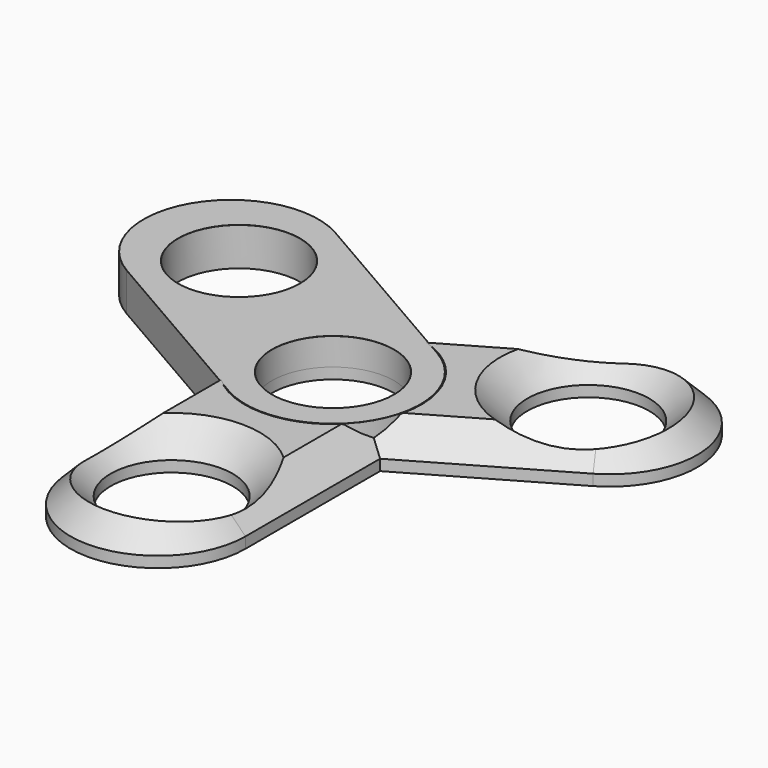
from build123d import *

# Parameters (mm, degrees)
F1_DEPTH    = 7
F2_R        = 11.15
F3_DEPTH    = 7.001
F5_COUNT    = 3
F6_R        = 0.0241421356
F7_T1_DEPTH = 40
F7_T3_DEPTH = 40
F7_T6_ANGLE = 180
F7_T8_ANGLE = 180
F8_T1_DEPTH = 40
F8_T4_ANGLE = 180
F8_T6_ANGLE = 180


# Not quite as in the source:
# - a fillet or chamfer that OpenCascade refuses, or shapes differently, is made with other operations: its cross-section is extruded or revolved along the edge and cut away or added


with BuildPart() as f1:
    # F0 (on Top) → F1 (new body)
    with BuildSketch(Plane.XY):
        with BuildLine():
            ThreePointArc((-16, 0), (0, -16), (16, 0))
            ThreePointArc((16, 0), (0, 16), (-16, 0))
        make_face()
        with BuildLine():
            Line((16, -40), (16, 0))
            ThreePointArc((16, 0), (0, -16), (-16, 0))
            Line((-16, 0), (-16, -40))
            ThreePointArc((-16, -40), (0, -24), (16, -40))
        make_face()
        with BuildLine():
            ThreePointArc((-16, -40), (0, -56), (16, -40))
            ThreePointArc((16, -40), (0, -24), (-16, -40))
        make_face()
    extrude(amount=F1_DEPTH)

    # F2 (on face) → F3 (cut, through all)
    with BuildSketch(Plane.XY.offset(7)):
        Circle(F2_R)
        with Locations((0, -36.8724052611)):
            Circle(F2_R)
    extrude(amount=-F3_DEPTH, mode=Mode.SUBTRACT)


with BuildPart() as f5_1:
    # F5: instance of F1
    add(f1.part.rotate(Axis((0, 0, -10.0436238572), (0, 0, -1)), 1 * 360 / F5_COUNT))

    # F6
    f6_edges = [f5_1.edges().sort_by_distance(p)[0] for p in [
        (-26.641016, 33.856406, 3.5),
        (13.856406, -8, 7),
        (-25.320508, -3.856406, 7),
        (-9.320508, 23.856406, 7),
        (-48.497423, 28, 7),
        (-26.35744, 28.092386, 7),
        (5.575, 9.656183, 7),
        (-42.641016, 6.143594, 3.5),
        (-8, -13.856406, 3.5),
        (-25.320508, -3.856406, 0),
        (-9.320508, 23.856406, 0),
    ]]
    fillet(f6_edges, radius=F6_R)


with BuildPart() as f5_2:
    # F5: instance of F1
    add(f1.part.rotate(Axis((0, 0, -10.0436238572), (0, 0, -1)), 2 * 360 / F5_COUNT))

    # F7: chamfer of 5 on 6 edges, made by hand

    # F7_s2 → F7_t1 (cut)
    with BuildSketch(Plane(origin=(34.6410161514, 20, 0), x_dir=(0, 0, 1), z_dir=(-0.8660254038, -0.5, 0))):
        Polygon((2, 16), (7, 11), (7, 16), align=None)
    extrude(amount=F7_T1_DEPTH, mode=Mode.SUBTRACT)

    # F7_s4 → F7_t3 (cut)
    with BuildSketch(Plane(origin=(0, 0, 0), x_dir=(0, 0, 1), z_dir=(0.8660254038, 0.5, 0))):
        Polygon((2, 16), (7, 11), (7, 16), align=None)
    extrude(amount=F7_T3_DEPTH, mode=Mode.SUBTRACT)

    # F7_s5 → F7_t6 (revolve, cut)
    with BuildSketch(Plane(origin=(0, 0, 0), x_dir=(0, 0, 1), z_dir=(0.8660254038, 0.5, 0))):
        Polygon((2, -16), (7, -11), (7, -16), align=None)
    revolve(axis=Axis((0, 0, 7), (0, 0, 1)), revolution_arc=F7_T6_ANGLE, mode=Mode.SUBTRACT)

    # F7_s7 → F7_t8 (revolve, cut)
    with BuildSketch(Plane(origin=(34.6410161514, 20, 0), x_dir=(0, 0, 1), z_dir=(-0.8660254038, -0.5, 0))):
        Polygon((7, -11), (2, -16), (7, -16), align=None)
    revolve(axis=Axis((34.6410161514, 20, 7), (0, 0, 1)), revolution_arc=F7_T8_ANGLE, mode=Mode.SUBTRACT)

    # F7_s9 → F7_t10 (revolve, cut)
    with BuildSketch(Plane(origin=(31.9324396547, 18.4362026305, 0), x_dir=(0, 0, 1), z_dir=(0.8660254038, 0.5, 0))):
        Polygon((7, -16.15), (2, -11.15), (7, -11.15), align=None)
    revolve(axis=Axis((31.9324396547, 18.4362026305, 7), (0, 0, 1)), mode=Mode.SUBTRACT)

    # F7_s11 → F7_t12 (revolve, cut)
    with BuildSketch(Plane(origin=(0, 0, 0), x_dir=(0, 0, 1), z_dir=(0.8660254038, 0.5, 0))):
        Polygon((7, -16.15), (2, -11.15), (7, -11.15), align=None)
    revolve(axis=Axis((0, 0, 7), (0, 0, 1)), mode=Mode.SUBTRACT)


with BuildPart() as f1_1:
    add(f1.part)

    # F8: chamfer of 5 on 6 edges, made by hand

    # F8_s2 → F8_t1 (cut)
    with BuildSketch(Plane.XZ):
        Polygon((16, 2), (11, 7), (16, 7), align=None)
        Polygon((-16, 2), (-11, 7), (-16, 7), align=None)
    extrude(amount=F8_T1_DEPTH, mode=Mode.SUBTRACT)

    # F8_s3 → F8_t4 (revolve, cut)
    with BuildSketch(Plane.XZ):
        Polygon((16, 2), (11, 7), (16, 7), align=None)
    revolve(axis=Axis((0, 0, 7), (0, 0, 1)), revolution_arc=F8_T4_ANGLE, mode=Mode.SUBTRACT)

    # F8_s5 → F8_t6 (revolve, cut)
    with BuildSketch(Plane.XZ.offset(40)):
        Polygon((-11, 7), (-16, 2), (-16, 7), align=None)
    revolve(axis=Axis((0, -40, 7), (0, 0, 1)), revolution_arc=F8_T6_ANGLE, mode=Mode.SUBTRACT)

    # F8_s7 → F8_t8 (revolve, cut)
    with BuildSketch(Plane.XZ.offset(36.8724052611)):
        Polygon((16.15, 7), (11.15, 2), (11.15, 7), align=None)
    revolve(axis=Axis((0, -36.8724052611, 7), (0, 0, 1)), mode=Mode.SUBTRACT)

    # F8_s9 → F8_t10 (revolve, cut)
    with BuildSketch(Plane.XZ):
        Polygon((16.15, 7), (11.15, 2), (11.15, 7), align=None)
    revolve(axis=Axis((0, 0, 7), (0, 0, 1)), mode=Mode.SUBTRACT)


solid = Compound([f5_1.part, f5_2.part, f1_1.part])
